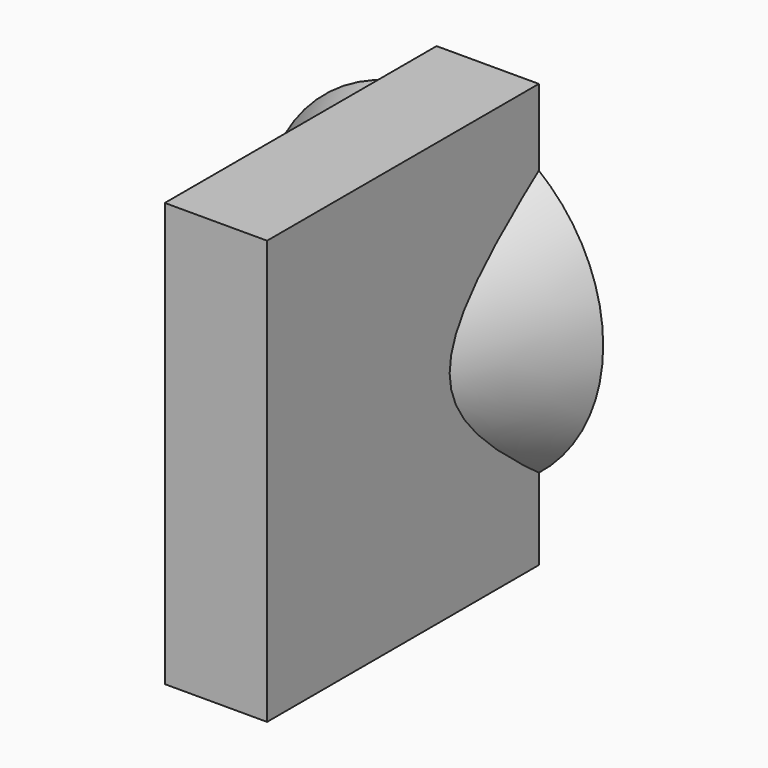
from build123d import *

# Parameters (mm, degrees)
F1_DEPTH  = 12.7
F1_TAPER  = 30
F1_FACE_R = 5.3676515813
F3_W      = 7.6477131806
F3_H      = 31.6800512373
F4_DEPTH  = 25.4
F6_DEPTH  = 0.508
F8_COUNT  = 20


# Not quite as in the source:
# - an extrude whose draft closes it to a point is written as a loft to that point


with BuildPart() as f1:
    # F0 (on Front) → F1 (new body)
    with BuildSketch(Plane.XZ):
        with BuildLine():
            ThreePointArc((-12.6853893316, 0.0378241174), (0.0146106684, -12.6621758826), (12.7146106684, 0.0378241174))
            Line((12.7146106684, 0.0378241174), (10.1746106684, 0.0378241174))
            ThreePointArc((10.1746106684, 0.0378241174), (0.0146106684, -10.1221758826), (-10.1453893316, 0.0378241174))
            Line((-10.1453893316, 0.0378241174), (-12.6853893316, 0.0378241174))
        make_face()
        with BuildLine():
            Line((10.1746106684, 0.0378241174), (12.7146106684, 0.0378241174))
            ThreePointArc((12.7146106684, 0.0378241174), (0.0146106684, 12.7378241174), (-12.6853893316, 0.0378241174))
            Line((-12.6853893316, 0.0378241174), (-10.1453893316, 0.0378241174))
            ThreePointArc((-10.1453893316, 0.0378241174), (0.0146106684, 10.1978241174), (10.1746106684, 0.0378241174))
        make_face()
        with BuildLine():
            Line((-10.1453893316, 0.0378241174), (10.1746106684, 0.0378241174))
            ThreePointArc((10.1746106684, 0.0378241174), (0.0146106684, 10.1978241174), (-10.1453893316, 0.0378241174))
        make_face()
        with BuildLine():
            ThreePointArc((-10.1453893316, 0.0378241174), (0.0146106684, -10.1221758826), (10.1746106684, 0.0378241174))
            Line((10.1746106684, 0.0378241174), (-10.1453893316, 0.0378241174))
        make_face()
    extrude(amount=F1_DEPTH, taper=F1_TAPER)

    # F1_face (on face) → F2 section 0
    with BuildSketch(Plane(origin=(0.0146106684, -12.7, 0.0378241174), x_dir=(1, 0, 0), z_dir=(0, -1, 0)), mode=Mode.PRIVATE) as f2_s0:
        Circle(F1_FACE_R)
    loft([f2_s0.sketch, Vertex(0.0146106684, -6.3030819442, 0.0378241174)], ruled=True, mode=Mode.SUBTRACT)


with BuildPart() as f4:
    # F3 (on Front) → F4 (new body)
    with BuildSketch(Plane.XZ):
        with Locations((4.0778565903, -0.1475326717)):
            Rectangle(F3_W, F3_H)
    extrude(amount=F4_DEPTH)


with BuildPart() as f6:
    # F5 (on face) → F6 (new body)
    with BuildSketch(Plane(origin=(0.254, 0, 0), x_dir=(0, -1, 0), z_dir=(-1, 0, 0))):
        Polygon((11.5401692409, -3.5125274417), (8.716051597, -1.1428113683), (8.2028126344, -1.7544657458), (10.9493458755, -4.0590807754), align=None)
    extrude(amount=F6_DEPTH)


with BuildPart() as f8_1:
    # F8: instance of F6
    add(f6.part.rotate(Axis((0, -10.6263123453, 0), (0, -1, 0)), 1 * 360 / F8_COUNT))


with BuildPart() as f8_2:
    # F8: instance of F6
    add(f6.part.rotate(Axis((0, -10.6263123453, 0), (0, -1, 0)), 2 * 360 / F8_COUNT))


with BuildPart() as f8_3:
    # F8: instance of F6
    add(f6.part.rotate(Axis((0, -10.6263123453, 0), (0, -1, 0)), 3 * 360 / F8_COUNT))


with BuildPart() as f8_4:
    # F8: instance of F6
    add(f6.part.rotate(Axis((0, -10.6263123453, 0), (0, -1, 0)), 4 * 360 / F8_COUNT))


with BuildPart() as f8_5:
    # F8: instance of F6
    add(f6.part.rotate(Axis((0, -10.6263123453, 0), (0, -1, 0)), 5 * 360 / F8_COUNT))


with BuildPart() as f8_6:
    # F8: instance of F6
    add(f6.part.rotate(Axis((0, -10.6263123453, 0), (0, -1, 0)), 6 * 360 / F8_COUNT))


with BuildPart() as f8_7:
    # F8: instance of F6
    add(f6.part.rotate(Axis((0, -10.6263123453, 0), (0, -1, 0)), 7 * 360 / F8_COUNT))


with BuildPart() as f8_8:
    # F8: instance of F6
    add(f6.part.rotate(Axis((0, -10.6263123453, 0), (0, -1, 0)), 8 * 360 / F8_COUNT))


with BuildPart() as f8_9:
    # F8: instance of F6
    add(f6.part.rotate(Axis((0, -10.6263123453, 0), (0, -1, 0)), 9 * 360 / F8_COUNT))


with BuildPart() as f8_10:
    # F8: instance of F6
    add(f6.part.rotate(Axis((0, -10.6263123453, 0), (0, -1, 0)), 10 * 360 / F8_COUNT))


with BuildPart() as f8_11:
    # F8: instance of F6
    add(f6.part.rotate(Axis((0, -10.6263123453, 0), (0, -1, 0)), 11 * 360 / F8_COUNT))


with BuildPart() as f8_12:
    # F8: instance of F6
    add(f6.part.rotate(Axis((0, -10.6263123453, 0), (0, -1, 0)), 12 * 360 / F8_COUNT))


with BuildPart() as f8_13:
    # F8: instance of F6
    add(f6.part.rotate(Axis((0, -10.6263123453, 0), (0, -1, 0)), 13 * 360 / F8_COUNT))


with BuildPart() as f8_14:
    # F8: instance of F6
    add(f6.part.rotate(Axis((0, -10.6263123453, 0), (0, -1, 0)), 14 * 360 / F8_COUNT))


with BuildPart() as f8_15:
    # F8: instance of F6
    add(f6.part.rotate(Axis((0, -10.6263123453, 0), (0, -1, 0)), 15 * 360 / F8_COUNT))


with BuildPart() as f8_16:
    # F8: instance of F6
    add(f6.part.rotate(Axis((0, -10.6263123453, 0), (0, -1, 0)), 16 * 360 / F8_COUNT))


with BuildPart() as f8_17:
    # F8: instance of F6
    add(f6.part.rotate(Axis((0, -10.6263123453, 0), (0, -1, 0)), 17 * 360 / F8_COUNT))


with BuildPart() as f8_18:
    # F8: instance of F6
    add(f6.part.rotate(Axis((0, -10.6263123453, 0), (0, -1, 0)), 18 * 360 / F8_COUNT))


with BuildPart() as f8_19:
    # F8: instance of F6
    add(f6.part.rotate(Axis((0, -10.6263123453, 0), (0, -1, 0)), 19 * 360 / F8_COUNT))


solid = Compound([f1.part, f4.part, f6.part, f8_1.part, f8_2.part, f8_3.part, f8_4.part, f8_5.part, f8_6.part, f8_7.part, f8_8.part, f8_9.part, f8_10.part, f8_11.part, f8_12.part, f8_13.part, f8_14.part, f8_15.part, f8_16.part, f8_17.part, f8_18.part, f8_19.part])
